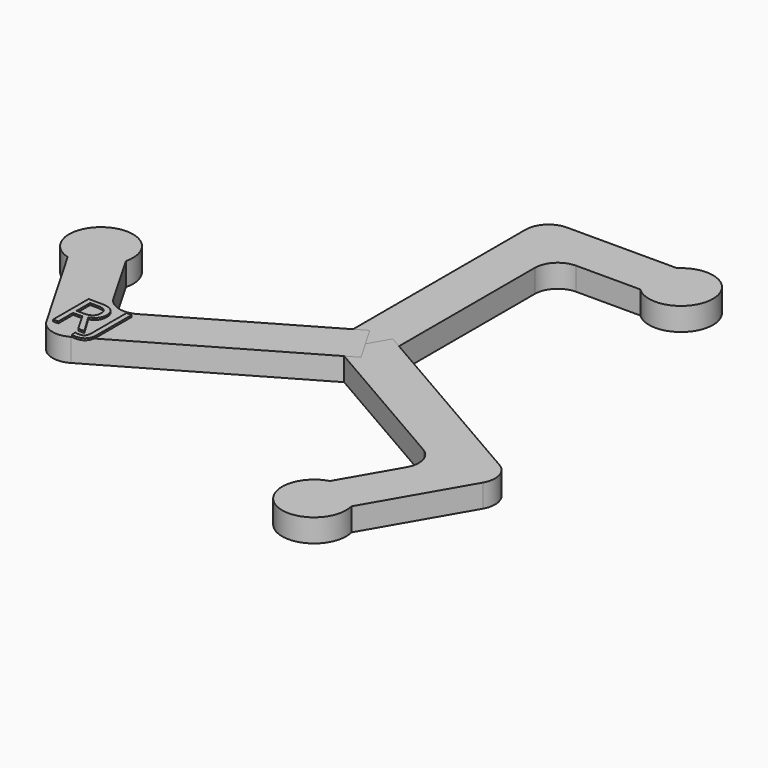
from build123d import *

# Parameters (mm, degrees)
F1_DEPTH     = 6.35
F3_COUNT     = 3
F4_TEXT_SIZE = 17.1263033014
F5_DEPTH     = 0.508


# Not quite as in the source:
# - Text() gives the source's letters only with a copy of the font that has no kerning and outlines rounded to 1/6400 em; it was checked with that copy


with BuildPart() as f1:
    # F0 (on Top) → F1 (new body)
    with BuildSketch(Plane.XY):
        with BuildLine():
            Line((12.7, 56.9171639323), (30.4464461657, 56.9171639323))
            ThreePointArc((30.4464461657, 56.9171639323), (45.437639544, 63.2671616449), (30.4464494517, 69.6171671152))
            Line((30.4464494517, 69.6171671152), (7.67e-08, 69.6171671152))
            ThreePointArc((7.67e-08, 69.6171671152), (-4.4901279838, 67.7572951757), (-6.3499999233, 63.2671671152))
            Line((-6.3499999233, 63.2671671152), (-6.3499999233, 0))
            Line((-6.3499999233, 0), (0, 0))
            Line((0, 0), (6.35, 0))
            Line((6.35, 0), (6.35, 50.5671639323))
            ThreePointArc((6.35, 50.5671639323), (8.2098719395, 55.0572919929), (12.7, 56.9171639323))
        make_face()
    extrude(amount=F1_DEPTH)


with BuildPart() as f3_1:
    # F3: instance of F1
    add(f1.part.rotate(Axis((0, 0, 12.816417031), (0, 0, -1)), 1 * 360 / F3_COUNT))


with BuildPart() as f3_2:
    # F3: instance of F1
    add(f1.part.rotate(Axis((0, 0, 12.816417031), (0, 0, -1)), 2 * 360 / F3_COUNT))

    # F4 (on face) → F5 (join)
    with BuildSketch(Plane.XY.offset(6.35)):
        with Locations((-60.7920385397, -33.939434784)):
            Text('RJ', F4_TEXT_SIZE, font='Open Sans', text_align=(TextAlign.LEFT, TextAlign.BOTTOM))
    extrude(amount=F5_DEPTH)


solid = Compound([f1.part, f3_1.part, f3_2.part])
